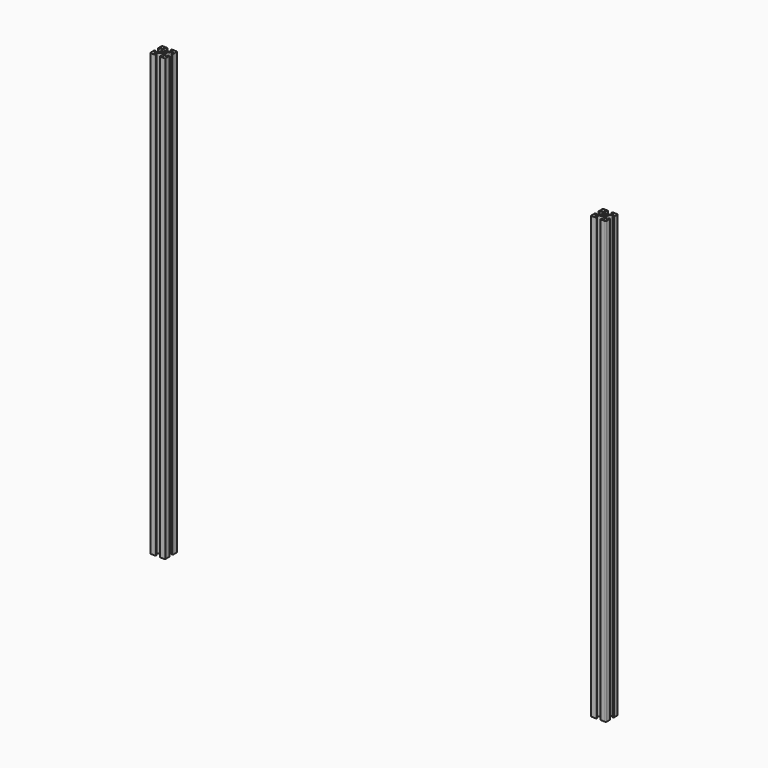
from build123d import *

# Parameters (mm, degrees)
F0_R     = 2.6035
F1_DEPTH = 736.6
F2_R     = 1.18109
F3_R     = 5.08
F4_R     = 0.762
F5_R     = 1.27


# Not quite as in the source:
# - a fillet or chamfer is up to 0.001 mm smaller than in the source, because OpenCascade refuses the exact size


with BuildPart() as f1:
    # F0 (on Top) → F1 (new body)
    with BuildSketch(Plane.XY):
        Polygon((12.7, 3.2385), (12.7, 12.7), (3.2385, 12.7), (3.2385, 10.3378), (8.7752354349, 10.3378), (2.9459354349, 4.5085), (-2.9459354349, 4.5085), (-8.7752354349, 10.3378), (-3.2385, 10.3378), (-3.2385, 12.7), (-12.7, 12.7), (-12.7, 3.2385), (-10.3378, 3.2385), (-10.3378, 8.7752354349), (-4.5085, 2.9459354349), (-4.5085, -2.9459354349), (-10.3378, -8.7752354349), (-10.3378, -3.2385), (-12.7, -3.2385), (-12.7, -12.7), (-3.2385, -12.7), (-3.2385, -10.3378), (-8.7752354349, -10.3378), (-2.9459354349, -4.5085), (2.9459354349, -4.5085), (8.7752354349, -10.3378), (3.2385, -10.3378), (3.2385, -12.7), (12.7, -12.7), (12.7, -3.2385), (10.3378, -3.2385), (10.3378, -8.7752354349), (4.5085, -2.9459354349), (4.5085, 2.9459354349), (10.3378, 8.7752354349), (10.3378, 3.2385), align=None)
        Circle(F0_R, mode=Mode.SUBTRACT)
    extrude(amount=F1_DEPTH)

    # F2 (radius 1.1811 in the source; OpenCascade refuses exactly that, so slightly less here)
    f2_edges = [f1.edges().sort_by_distance(p)[0] for p in [
        (3.2385, 12.7, 368.3),
        (3.2385, 10.3378, 368.3),
        (-3.2385, 12.7, 368.3),
        (-12.7, 3.2385, 368.3),
        (-3.2385, 10.3378, 368.3),
        (-10.3378, 3.2385, 368.3),
        (12.7, 3.2385, 368.3),
        (10.3378, 3.2385, 368.3),
        (12.7, -3.2385, 368.3),
        (10.3378, -3.2385, 368.3),
        (3.2385, -10.3378, 368.3),
        (-3.2385, -10.3378, 368.3),
        (-10.3378, -3.2385, 368.3),
        (-12.7, -3.2385, 368.3),
        (-3.2385, -12.7, 368.3),
        (3.2385, -12.7, 368.3),
    ]]
    fillet(f2_edges, radius=F2_R)

    # F3
    f3_edges = [f1.edges().sort_by_distance(p)[0] for p in [
        (2.945935, 4.5085, 368.3),
        (-2.945935, 4.5085, 368.3),
        (4.5085, -2.945935, 368.3),
        (4.5085, 2.945935, 368.3),
        (2.945935, -4.5085, 368.3),
        (-2.945935, -4.5085, 368.3),
        (-4.5085, -2.945935, 368.3),
        (-4.5085, 2.945935, 368.3),
    ]]
    fillet(f3_edges, radius=F3_R)

    # F4
    f4_edges = [f1.edges().sort_by_distance(p)[0] for p in [
        (8.775235, 10.3378, 368.3),
        (-8.775235, 10.3378, 368.3),
        (-10.3378, 8.775235, 368.3),
        (-10.3378, -8.775235, 368.3),
        (-8.775235, -10.3378, 368.3),
        (8.775235, -10.3378, 368.3),
        (10.3378, -8.775235, 368.3),
        (10.3378, 8.775235, 368.3),
    ]]
    fillet(f4_edges, radius=F4_R)

    # F5
    f5_edges = [f1.edges().sort_by_distance(p)[0] for p in [
        (-12.7, -12.7, 368.3),
        (12.7, -12.7, 368.3),
        (12.7, 12.7, 368.3),
        (-12.7, 12.7, 368.3),
    ]]
    fillet(f5_edges, radius=F5_R)


with BuildPart() as f6_1:
    # F6: copy of F1
    add(f1.part.moved(Location((736.6, 0, 0))))


solid = Compound([f1.part, f6_1.part])
